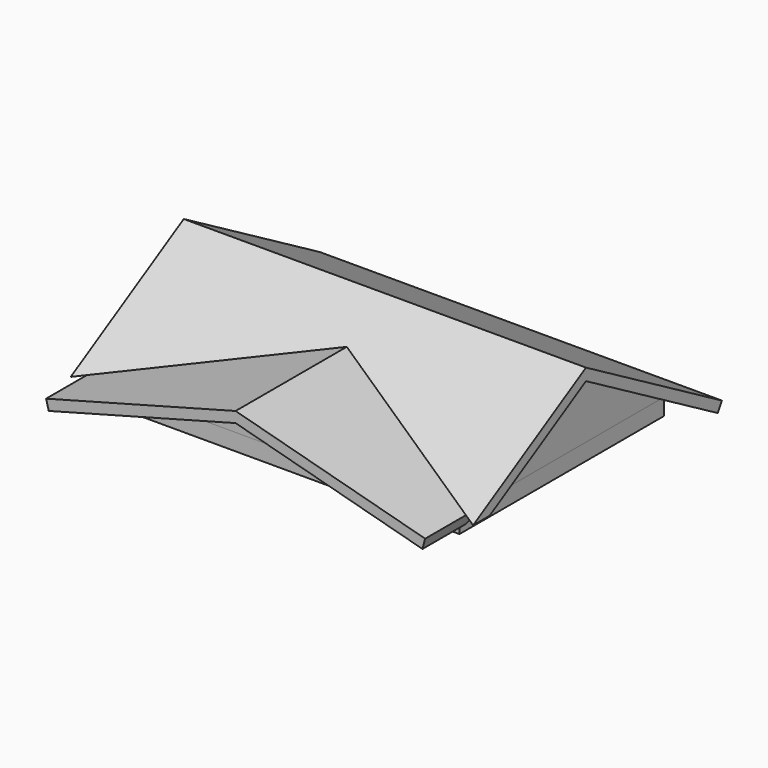
from build123d import *

# Parameters (mm, degrees)
F1_DEPTH       = 34
F3_DEPTH       = 770.75
F3_DEPTH_BACK  = 49.25
F4_DEPTH       = 21
F5_START       = -700.5
F5_DEPTH       = 21
F6_DEPTH       = 5
F8_DEPTH       = 21
F7_W           = 721.5
F7_H           = 34
F9_DEPTH       = 200
F9_DEPTH_BACK  = 50
F10_W          = 820
F10_H          = 41.1768076986
F11_DEPTH      = 50
F11_TAPER      = -3
F12_DEPTH      = 200
F12_DEPTH_BACK = 120
F14_DEPTH      = 300
F16_DEPTH      = 800


with BuildPart() as f1:
    # F0 (on Top) → F1 (new body)
    with BuildSketch(Plane.XY):
        Polygon((345.3741043846, -282.3741084489), (360.3741043846, -297.3741084489), (360.3741043846, 224.1258915511), (345.3741043846, 209.1258915511), align=None)
        Polygon((326.3741043846, -263.3741084489), (341.3741043846, -278.3741084489), (341.3741043846, 205.1258915511), (326.3741043846, 190.1258915511), align=None)
        Polygon((-346.1258956154, -282.3741084489), (-361.1258956154, -297.3741084489), (360.3741043846, -297.3741084489), (345.3741043846, -282.3741084489), align=None)
        Polygon((360.3741043846, 224.1258915511), (-361.1258956154, 224.1258915511), (-346.1258956154, 209.1258915511), (345.3741043846, 209.1258915511), align=None)
        Polygon((-361.1258956154, 224.1258915511), (-361.1258956154, -297.3741084489), (-346.1258956154, -282.3741084489), (-346.1258956154, 209.1258915511), align=None)
        Polygon((-327.1258956154, -263.3741084489), (-342.1258956154, -278.3741084489), (341.3741043846, -278.3741084489), (326.3741043846, -263.3741084489), align=None)
        Polygon((-342.1258956154, 205.1258915511), (-342.1258956154, -278.3741084489), (-327.1258956154, -263.3741084489), (-327.1258956154, 190.1258915511), align=None)
        Polygon((341.3741043846, 205.1258915511), (-342.1258956154, 205.1258915511), (-327.1258956154, 190.1258915511), (326.3741043846, 190.1258915511), align=None)
        Polygon((341.3741043846, -278.3741084489), (345.3741043846, -282.3741084489), (345.3741043846, 209.1258915511), (341.3741043846, 205.1258915511), align=None)
        Polygon((-342.1258956154, -278.3741084489), (-346.1258956154, -282.3741084489), (345.3741043846, -282.3741084489), (341.3741043846, -278.3741084489), align=None)
        Polygon((-346.1258956154, 209.1258915511), (-346.1258956154, -282.3741084489), (-342.1258956154, -278.3741084489), (-342.1258956154, 205.1258915511), align=None)
        Polygon((345.3741043846, 209.1258915511), (-346.1258956154, 209.1258915511), (-342.1258956154, 205.1258915511), (341.3741043846, 205.1258915511), align=None)
    extrude(amount=F1_DEPTH)

    # F0 (on Top) → F6 (cut)
    with BuildSketch(Plane.XY):
        Polygon((345.3741043846, 209.1258915511), (-346.1258956154, 209.1258915511), (-342.1258956154, 205.1258915511), (341.3741043846, 205.1258915511), align=None)
        Polygon((-346.1258956154, 209.1258915511), (-346.1258956154, -282.3741084489), (-342.1258956154, -278.3741084489), (-342.1258956154, 205.1258915511), align=None)
        Polygon((-342.1258956154, -278.3741084489), (-346.1258956154, -282.3741084489), (345.3741043846, -282.3741084489), (341.3741043846, -278.3741084489), align=None)
        Polygon((341.3741043846, -278.3741084489), (345.3741043846, -282.3741084489), (345.3741043846, 209.1258915511), (341.3741043846, 205.1258915511), align=None)
    extrude(amount=F6_DEPTH, mode=Mode.SUBTRACT)


with BuildPart() as f3:
    # F2 (on face) → F3 (new body, two sides)
    with BuildSketch(Plane(origin=(-361.1258956154, 0, 0), x_dir=(0, -1, 0), z_dir=(-1, 0, 0))) as f3_sk:
        Polygon((-224.1258915511, 34), (36.6241084489, 184.5440826912), (36.6241084489, 208.7927939972), (-309.7860530649, 8.7927939972), (-299.2860530649, -9.3937394823), align=None)
        Polygon((36.6241084489, 208.7927939972), (36.6241084489, 184.5440826912), (276.3741084489, 46.124355653), (297.3741084489, 34), (372.5342699626, -9.3937394823), (383.0342699626, 8.7927939972), align=None)
    extrude(amount=-F3_DEPTH)
    extrude(f3_sk.sketch, amount=F3_DEPTH_BACK)

    # F7 (on face) → F9 (cut, two sides)
    with BuildSketch(Plane.XZ.offset(297.3741084489)) as f9_sk:
        Polygon((-361.1258956154, 0), (-361.1258956154, 34), (-380.9351305685, 28.6921314917), (-386.3703305156, 48.9765738437), (-569.1533924811, 0), align=None)
        Polygon((-380.9351305685, 28.6921314917), (-361.1258956154, 34), (0, 130.7633920961), (0, 152.5041918847), (-386.3703305156, 48.9765738437), align=None)
        Polygon((361.1258956154, 34), (360.3741043846, 34), (360.3741043846, 0), (569.1533924811, 0), (386.3703305156, 48.9765738437), (380.9351305685, 28.6921314917), align=None)
        Polygon((0, 152.5041918847), (0, 130.7633920961), (361.1258956154, 34), (380.9351305685, 28.6921314917), (386.3703305156, 48.9765738437), align=None)
        Polygon((0, 130.7633920961), (-361.1258956154, 34), (360.3741043846, 34), (361.1258956154, 34), align=None)
        with Locations((-0.3758956154, 17)):
            Rectangle(F7_W, F7_H)
    extrude(amount=-F9_DEPTH, mode=Mode.SUBTRACT)
    extrude(f9_sk.sketch, amount=F9_DEPTH_BACK, mode=Mode.SUBTRACT)

    # F10 (on face) → F11 (cut)
    with BuildSketch(Plane(origin=(0, -99.5659589765, 172.4532996517), x_dir=(1, 0, 0), z_dir=(0, -0.5, 0.8660254038))):
        Polygon((409.6241043846, -259.4151114743), (0, -39.8982155339), (-410.3758956154, -259.8179951806), (-612.6573998522, -368.2203265886), (612.6573998522, -368.2203265886), align=None)
        with Locations((-0.3758956154, -306.7326074598)):
            Rectangle(F10_W, F10_H, mode=Mode.SUBTRACT)
        with Locations((-0.3758956154, -306.7326074598)):
            Rectangle(F10_W, F10_H)
    extrude(amount=-F11_DEPTH, taper=F11_TAPER, mode=Mode.SUBTRACT)


with BuildPart() as f4:
    # F2 (on face) → F4 (new body)
    with BuildSketch(Plane(origin=(-361.1258956154, 0, 0), x_dir=(0, -1, 0), z_dir=(-1, 0, 0))):
        Polygon((-203.1258915511, 34), (36.6241084489, 34), (36.6241084489, 184.5440826912), (-224.1258915511, 34), align=None)
        Polygon((36.6241084489, 184.5440826912), (36.6241084489, 34), (276.3741084489, 34), (276.3741084489, 46.124355653), align=None)
    extrude(amount=-F4_DEPTH)


with BuildPart() as f5:
    # F2 (on face) → F5 (new body)
    with BuildSketch(Plane(origin=(-361.1258956154, 0, 0), x_dir=(0, -1, 0), z_dir=(-1, 0, 0)).offset(F5_START)):
        Polygon((-203.1258915511, 34), (36.6241084489, 34), (36.6241084489, 184.5440826912), (-224.1258915511, 34), align=None)
        Polygon((36.6241084489, 184.5440826912), (36.6241084489, 34), (276.3741084489, 34), (276.3741084489, 46.124355653), align=None)
    extrude(amount=-F5_DEPTH)


with BuildPart() as f8:
    # F7 (on face) → F8 (new body)
    with BuildSketch(Plane.XZ.offset(297.3741084489)):
        Polygon((0, 130.7633920961), (-361.1258956154, 34), (360.3741043846, 34), (361.1258956154, 34), align=None)
    extrude(amount=-F8_DEPTH)


with BuildPart() as f12:
    # F7 (on face) → F12 (new body, two sides)
    with BuildSketch(Plane.XZ.offset(297.3741084489)) as f12_sk:
        Polygon((0, 152.5041918847), (0, 130.7633920961), (361.1258956154, 34), (380.9351305685, 28.6921314917), (386.3703305156, 48.9765738437), align=None)
        Polygon((-380.9351305685, 28.6921314917), (-361.1258956154, 34), (0, 130.7633920961), (0, 152.5041918847), (-386.3703305156, 48.9765738437), align=None)
    extrude(amount=-F12_DEPTH)
    extrude(f12_sk.sketch, amount=F12_DEPTH_BACK)

    # F13 (on face) → F14 (cut)
    with BuildSketch(Plane(origin=(0, -89.0659589765, 154.2667661722), x_dir=(1, 0, 0), z_dir=(0, 0.5, -0.8660254038))):
        Polygon((-410.3758956154, -60.5546330379), (409.6241043846, -60.5546330379), (409.6241043846, 223.0420445153), (11.3235573479, 9.5934246686), (-11.3235573479, 9.5934246686), (-410.3758956154, 223.4449282217), align=None)
    extrude(amount=F14_DEPTH, mode=Mode.SUBTRACT)

    # F15 (on face) → F16 (cut)
    with BuildSketch(Plane.YZ.offset(409.6241043846)):
        Polygon((-24.5864332149, 127.3517449025), (-52.3608607368, 175.4584645216), (-282.2260356388, 42.7457439146), (-409.6211082826, -30.8058355697), (-403.7217834932, -91.54215164), align=None)
    extrude(amount=-F16_DEPTH, mode=Mode.SUBTRACT)


solid = Compound([f1.part, f3.part, f4.part, f5.part, f8.part, f12.part])
